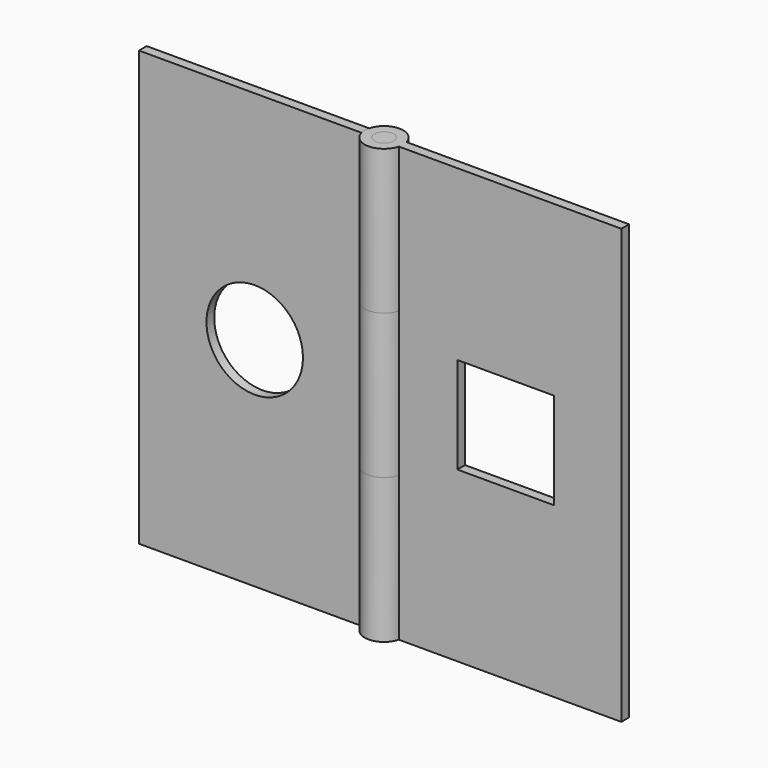
from build123d import *

# Parameters (mm, degrees)
F0_R      = 2
F1_DEPTH  = 45
F2_DEPTH  = 45
F3_DEPTH  = 15
F4_DEPTH  = 45
F5_DEPTH  = 30
F6_DEPTH  = 30
F7_R      = 10
F8_DEPTH  = 5.001
F9_W      = 20
F9_H      = 20
F10_DEPTH = 5.001


with BuildPart() as f1:
    # F0 (on Top) → F1 (new body, symmetric)
    with BuildSketch(Plane.XY):
        Circle(F0_R)
    extrude(amount=F1_DEPTH, both=True)


with BuildPart() as f2:
    # F0 (on Top) → F2 (new body, symmetric)
    with BuildSketch(Plane.XY):
        with BuildLine():
            ThreePointArc((-3.8729833462, -1), (-4, 0), (-3.8729833462, 1))
            Line((-3.8729833462, 1), (-50, 1))
            Line((-50, 1), (-50, -1))
            Line((-50, -1), (-3.8729833462, -1))
        make_face()
    extrude(amount=F2_DEPTH, both=True)

    # F0 (on Top) → F3 (join, symmetric)
    with BuildSketch(Plane.XY):
        with BuildLine():
            ThreePointArc((3.8729833462, -1), (3.9681187851, -0.5040171699), (4, 0))
            ThreePointArc((4, 0), (3.9681187851, 0.5040171699), (3.8729833462, 1))
            ThreePointArc((3.8729833462, 1), (0, 4), (-3.8729833462, 1))
            ThreePointArc((-3.8729833462, 1), (-4, 0), (-3.8729833462, -1))
            ThreePointArc((-3.8729833462, -1), (0, -4), (3.8729833462, -1))
        make_face()
        Circle(F0_R, mode=Mode.SUBTRACT)
    extrude(amount=F3_DEPTH, both=True)


with BuildPart() as f4:
    # F0 (on Top) → F4 (new body, symmetric)
    with BuildSketch(Plane.XY):
        with BuildLine():
            ThreePointArc((3.8729833462, 1), (3.9681187851, 0.5040171699), (4, 0))
            ThreePointArc((4, 0), (3.9681187851, -0.5040171699), (3.8729833462, -1))
            Line((3.8729833462, -1), (50, -1))
            Line((50, -1), (50, 1))
            Line((50, 1), (3.8729833462, 1))
        make_face()
    extrude(amount=F4_DEPTH, both=True)

    # F5 (add, through all): a face of the model
    f5_faces = [f2.part.faces().sort_by_distance(p)[0] for p in [
        (-3.886862915, 0, 15),
    ]]
    extrude(f5_faces, amount=F5_DEPTH)

    # F6 (add, through all): a face of the model
    f6_faces = [f2.part.faces().sort_by_distance(p)[0] for p in [
        (-3.886862915, 0, -15),
    ]]
    extrude(f6_faces, amount=F6_DEPTH)

    # F9 (on face) → F10 (cut, through all)
    with BuildSketch(Plane.XZ.offset(1)):
        with Locations((26, 0)):
            Rectangle(F9_W, F9_H)
    extrude(amount=-F10_DEPTH, mode=Mode.SUBTRACT)


with BuildPart() as f2_1:
    add(f2.part)

    # F7 (on face) → F8 (cut, through all)
    with BuildSketch(Plane.XZ.offset(1)):
        with Locations((-26, 0)):
            Circle(F7_R)
    extrude(amount=-F8_DEPTH, mode=Mode.SUBTRACT)


solid = Compound([f1.part, f4.part, f2_1.part])
